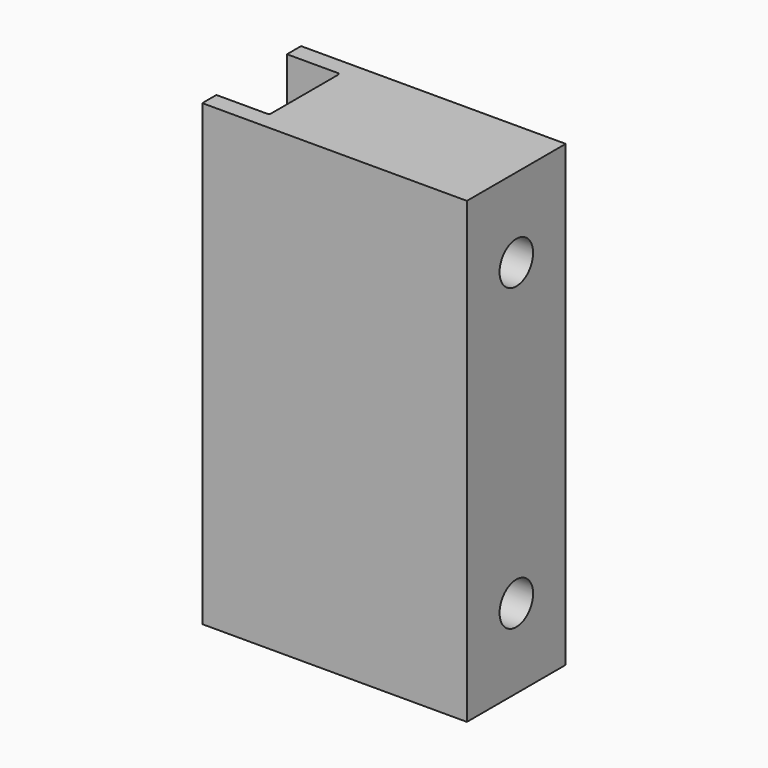
from build123d import *

# Parameters (mm, degrees)
F1_DEPTH       = 165.1
F3_D           = 20.6375
F3_CBORE_D     = 30.1752
F3_CBORE_DEPTH = 28.448
F4_R           = 1.524


# Not quite as in the source:
# - a length typed as a fraction of an inch, garbled in the dataset ("3 / 203.2 mm" for 3/8 in), is restored


with BuildPart() as f1:
    # F0 (on Top) → F1 (new body, symmetric)
    with BuildSketch(Plane.XY):
        Polygon((95.25, 44.45), (-95.25, 44.45), (-95.25, 31.75), (-57.15, 31.75), (-57.15, -31.75), (-95.25, -31.75), (-95.25, -44.45), (95.25, -44.45), align=None)
    extrude(amount=F1_DEPTH, both=True)

    # F3 (through all)
    with Locations(Plane.YZ.offset(95.25)):
        with Locations((0, 107.95), (0, -107.95)):
            CounterBoreHole(F3_D / 2, F3_CBORE_D / 2, F3_CBORE_DEPTH)

    # F4
    f4_edges = [f1.edges().sort_by_distance(p)[0] for p in [
        (-57.15, 31.75, 0),
        (-57.15, -31.75, 0),
    ]]
    fillet(f4_edges, radius=F4_R)


solid = f1.part
